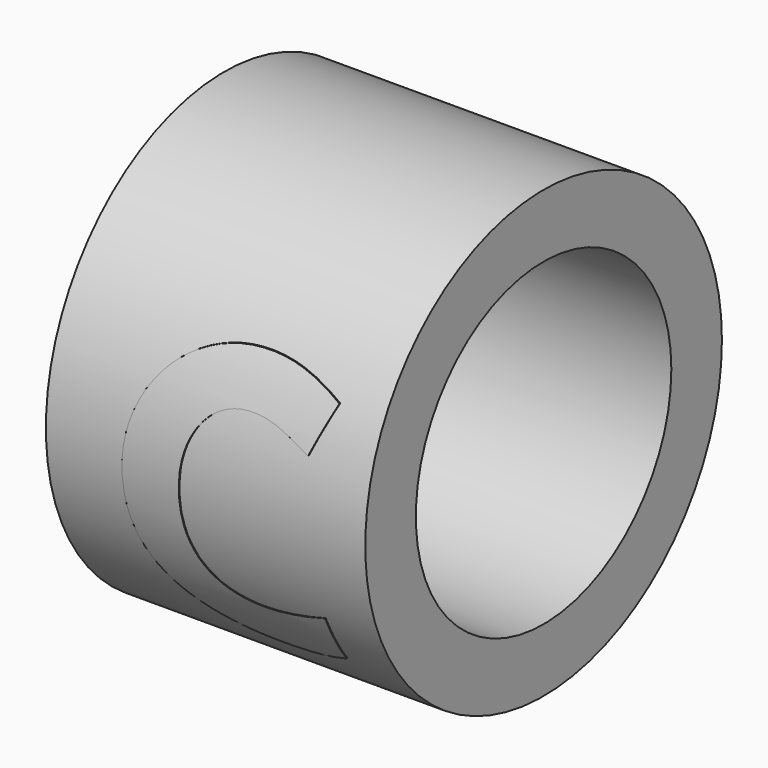
from build123d import *

# Parameters (mm, degrees)
F0_R         = 1.75
F0_R_2       = 1.745
F0_R_3       = 1.25
F1_DEPTH     = 2.5
F2_TEXT_SIZE = 2.8570699214
F3_REACH     = 4.3608869614
F4_DEPTH     = 2.5


# Not quite as in the source:
# - Text() gives the source's letters only with a copy of the font that has no kerning and outlines rounded to 1/6400 em; it was checked with that copy


with BuildPart() as f1:
    # F0 (on Right) → F1 (new body)
    with BuildSketch(Plane.YZ):
        Circle(F0_R)
        Circle(F0_R_2, mode=Mode.SUBTRACT)
        Circle(F0_R_2)
        Circle(F0_R_3, mode=Mode.SUBTRACT)
    extrude(amount=F1_DEPTH)

    f3_end = f1.faces().sort_by_distance((1.25, -1.75, 0))[0]
    # F2 (on Front) → F3 (intersect, up to a face of the model that its end follows)
    with BuildSketch(Plane.XZ):
        with Locations((0.4309935612, -1.1343103251)):
            Text('C', F2_TEXT_SIZE, font='Open Sans', font_style=FontStyle.BOLD, text_align=(TextAlign.LEFT, TextAlign.BOTTOM))
    f3_long = extrude(amount=F3_REACH, mode=Mode.PRIVATE)
    add(split(f3_long, bisect_by=f3_end, keep=Keep.BOTTOM, mode=Mode.PRIVATE), mode=Mode.INTERSECT)


with BuildPart() as f4:
    # F0 (on Right) → F4 (new body)
    with BuildSketch(Plane.YZ):
        Circle(F0_R_2)
        Circle(F0_R_3, mode=Mode.SUBTRACT)
    extrude(amount=F4_DEPTH)


solid = Compound([f1.part, f4.part])
